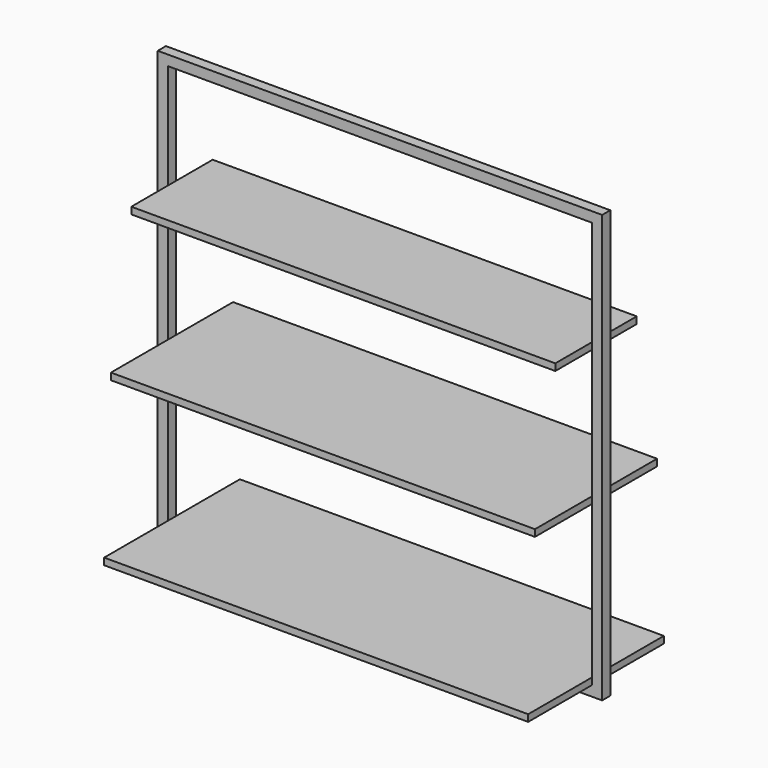
from build123d import *

# Parameters (mm, degrees)
F0_W     = 1250
F0_H     = 500
F1_DEPTH = 20
F2_W     = 1310
F2_H     = 1260
F2_W_2   = 1250
F2_H_2   = 1200
F3_DEPTH = 15
F4_W     = 1050
F4_H     = 300
F4_W_2   = 990
F4_H_2   = 240
F5_DEPTH = 30
F6_W     = 1250
F6_H     = 20
F7_DEPTH = 150
F8_W     = 1250
F8_H     = 20
F9_DEPTH = 225


with BuildPart() as f1:
    # F0 (on Top) → F1 (new body)
    with BuildSketch(Plane.XY):
        Rectangle(F0_W, F0_H)
    extrude(amount=F1_DEPTH)


with BuildPart() as f3:
    # F2 (on Front) → F3 (new body, symmetric)
    with BuildSketch(Plane.XZ):
        with Locations((0, 600)):
            Rectangle(F2_W, F2_H)
        with Locations((0, 600)):
            Rectangle(F2_W_2, F2_H_2, mode=Mode.SUBTRACT)
    extrude(amount=F3_DEPTH, both=True)

    # F4 (on face) → F5 (join)
    with BuildSketch(Plane(origin=(0, 0, 0), x_dir=(1, 0, 0), z_dir=(0, 0, -1))):
        Rectangle(F4_W, F4_H)
        Rectangle(F4_W_2, F4_H_2, mode=Mode.SUBTRACT)
    extrude(amount=F5_DEPTH)


with BuildPart() as f7:
    # F6 (on Front) → F7 (new body, symmetric)
    with BuildSketch(Plane.XZ):
        with Locations((0, 880)):
            Rectangle(F6_W, F6_H)
    extrude(amount=F7_DEPTH, both=True)


with BuildPart() as f9:
    # F8 (on Front) → F9 (new body, symmetric)
    with BuildSketch(Plane.XZ):
        with Locations((0, 480)):
            Rectangle(F8_W, F8_H)
    extrude(amount=F9_DEPTH, both=True)


solid = Compound([f1.part, f3.part, f7.part, f9.part])
